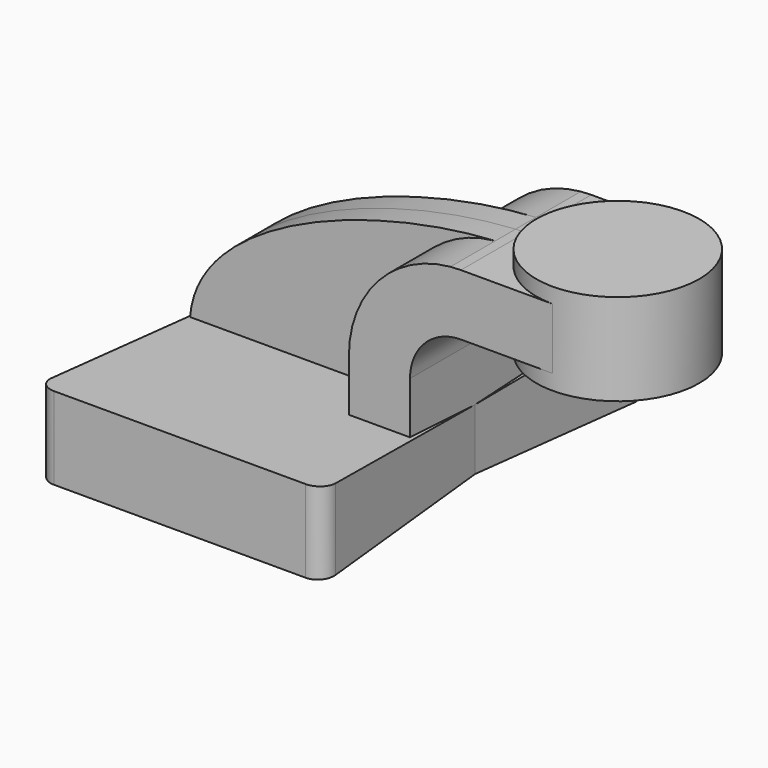
from build123d import *

# Parameters (mm, degrees)
F1_DEPTH = 63.5
F1_TAPER = -3
F0_W     = 25.4
F0_H     = 19.05
F2_DEPTH = 25.4
F3_DEPTH = 7.9375
F5_R     = 5.08


with BuildPart() as f1:
    # F0 (on Front) → F1 (new body, symmetric)
    with BuildSketch(Plane.XZ):
        Polygon((22.225, 9.525), (-41.275, 9.525), (-41.275, -9.525), (41.275, -9.525), (41.275, 9.525), align=None)
    extrude(amount=F1_DEPTH, both=True, taper=F1_TAPER)

    # F0 (on Front) → F2 (join, symmetric)
    with BuildSketch(Plane.XZ):
        with BuildLine():
            Line((22.225, 27.0002), (22.225, 9.525))
            Line((22.225, 9.525), (41.275, 9.525))
            Line((41.275, 9.525), (41.275, 27.0002))
            ThreePointArc((41.275, 27.0002), (45.9246798487, 38.2255201513), (57.15, 42.8752))
            Line((57.15, 42.8752), (60.325, 42.8752))
            Line((60.325, 42.8752), (60.325, 61.9252))
            Line((60.325, 61.9252), (57.15, 61.9252))
            add(Edge.make_bspline(
                [(53.8854342407, 61.7722898912), (54.9842067368, 61.8365871986), (56.0728453275, 61.8876096574), (57.15, 61.9252)],
                knots=[108.5245810491, 108.5245810491, 108.5245810491, 108.5245810491, 111.5045361635, 111.5045361635, 111.5045361635, 111.5045361635], degree=3))
            ThreePointArc((53.8854342407, 61.7722898912), (31.3258777096, 50.5133948686), (22.225, 27.0002))
        make_face()
        with Locations((73.025, 52.4002)):
            Rectangle(F0_W, F0_H)
    extrude(amount=F2_DEPTH, both=True)

    # F0 (on Front) → F3 (join, symmetric)
    with BuildSketch(Plane.XZ):
        with BuildLine():
            add(Edge.make_bspline(
                [(-41.275, 9.525), (-39.5856284224, 39.4828766469), (13.870125209, 59.4306981306), (53.8854342407, 61.7722898912)],
                knots=[0, 0, 0, 0, 108.5245810491, 108.5245810491, 108.5245810491, 108.5245810491], degree=3))
            Line((-41.275, 9.525), (22.225, 9.525))
            Line((22.225, 9.525), (22.225, 27.0002))
            ThreePointArc((22.225, 27.0002), (31.3258777096, 50.5133948686), (53.8854342407, 61.7722898912))
        make_face()
    extrude(amount=F3_DEPTH, both=True)

    # F0 (on Front) → F4 (revolve)
    with BuildSketch(Plane.XZ):
        Polygon((85.725, 66.675), (85.725, 61.9252), (85.725, 42.8752), (85.725, 38.1), (111.125, 38.1), (111.125, 66.675), align=None)
    revolve(axis=Axis((85.725, 0, 52.3875), (0, 0, 1)))

    # F5
    f5_edges = [f1.edges().sort_by_distance(p)[0] for p in [
        (44.602894, -63.5, 0),
        (-44.602894, -63.5, 0),
        (44.602894, 63.5, 0),
        (-44.602894, 63.5, 0),
    ]]
    fillet(f5_edges, radius=F5_R)


solid = f1.part
